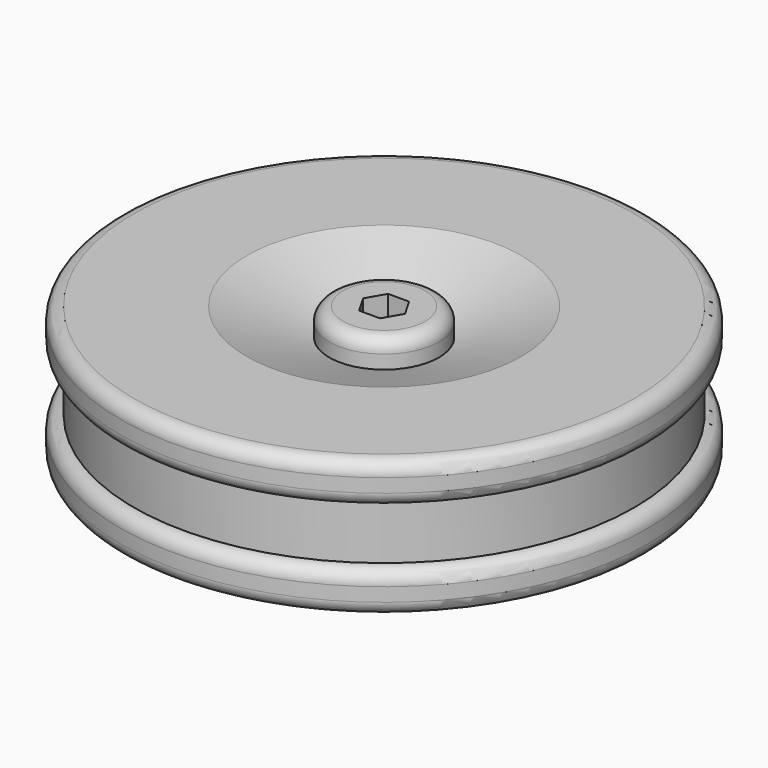
from build123d import *

# Parameters (mm, degrees)
F0_R      = 19.25
F0_R_2    = 1
F1_DEPTH  = 10
F4_R      = 10
F3_R      = 4
F8_R      = 10
F7_R      = 4
F11_R     = 4
F11_R_2   = 1
F12_DEPTH = 2
F14_R     = 19.25
F14_R_2   = 18.25
F15_DEPTH = 4
F16_R     = 0.99999
F18_DEPTH = 25


# Not quite as in the source:
# - a fillet or chamfer is up to 0.001 mm smaller than in the source, because OpenCascade refuses the exact size
# - a feature of the source that left no trace in its solid (it failed there, or was rolled back) is left out
# - a pattern or mirror of a feature is missing from the dataset's text; its kind, count and spacing are read off the source's solid


with BuildPart() as f1:
    # F0 (on Top) → F1 (new body)
    with BuildSketch(Plane.XY):
        Circle(F0_R)
        Circle(F0_R_2, mode=Mode.SUBTRACT)
    extrude(amount=F1_DEPTH)

    # F4 (on face) → F5 section 0
    with BuildSketch(Plane.XY.offset(10)):
        Circle(F4_R)
    # F3 (on offset) → F5 section 1
    with BuildSketch(Plane.XY.offset(8)):
        Circle(F3_R)
    loft(mode=Mode.SUBTRACT)

    # F8 (on face) → F9 section 0
    with BuildSketch(Plane.XY):
        Circle(F8_R)
    # F7 (on offset) → F9 section 1
    with BuildSketch(Plane.XY.offset(2)):
        Circle(F7_R)
    loft(mode=Mode.SUBTRACT)

    # F11 (on face) → F12 (join, through all)
    with BuildSketch(Plane.XY):
        Circle(F11_R)
        Circle(F11_R_2, mode=Mode.SUBTRACT)
    f12 = extrude(amount=F12_DEPTH)

    # F12_copies: F12 across plane
    add(f12.mirror(Plane.XY.offset(5)))

    # F14 (on offset) → F15 (cut)
    with BuildSketch(Plane.XY.offset(3)):
        Circle(F14_R)
        Circle(F14_R_2, mode=Mode.SUBTRACT)
    extrude(amount=F15_DEPTH, mode=Mode.SUBTRACT)

    # F16 (radius 1 in the source; OpenCascade refuses exactly that, so slightly less here)
    f16_edges = [f1.edges().sort_by_distance(p)[0] for p in [
        (-4, 0, 0),
        (-19.25, 0, 10),
        (-19.25, 0, 0),
        (-19.25, 0, 7),
        (-19.25, 0, 3),
        (-4, 0, 10),
    ]]
    fillet(f16_edges, radius=F16_R)

    # F17 (on Top) → F18 (cut)
    with BuildSketch(Plane.XY):
        Polygon((0.7649891067, 1.325), (-0.7649891067, 1.325), (-1.5299782134, 0), (-0.7649891067, -1.325), (0.7649891067, -1.325), (1.5299782134, 0), align=None)
    extrude(amount=F18_DEPTH, mode=Mode.SUBTRACT)


solid = f1.part
